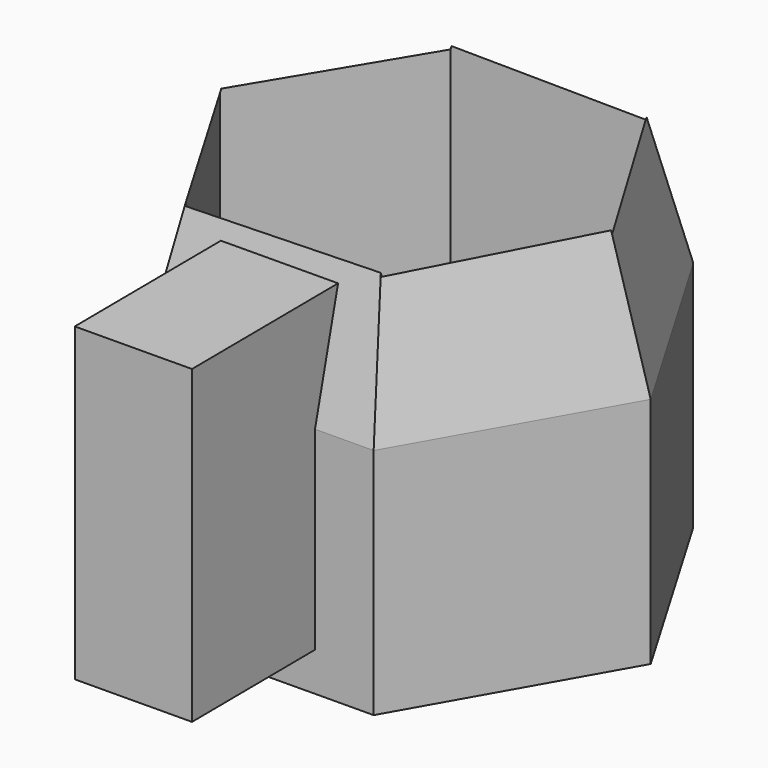
from build123d import *

# Parameters (mm, degrees)
F1_DEPTH     = 50
F3_DEPTH     = 45
F4_W         = 15
F4_H         = 40
F5_DEPTH     = 20
F6_T1_DEPTH  = 133.8850999909
F6_T3_DEPTH  = 133.8850999909
F6_T5_DEPTH  = 133.8850999909
F6_T10_DEPTH = 133.8850999909
F6_T15_DEPTH = 133.8850999909
F6_T20_DEPTH = 133.8850999909
F6_T25_DEPTH = 133.8850999909
F6_T30_DEPTH = 133.8850999909


# Not quite as in the source:
# - a fillet or chamfer that OpenCascade refuses, or shapes differently, is made with other operations: its cross-section is extruded or revolved along the edge and cut away or added


with BuildPart() as f1:
    # F0 (on Top) → F1 (new body)
    with BuildSketch(Plane.XY):
        Polygon((29.9990277389, 0.2415258118), (14.7903463808, 26.1006830166), (-15.2086813581, 25.8591572049), (-29.9990277389, -0.2415258118), (-14.7903463808, -26.1006830166), (15.2086813581, -25.8591572049), align=None)
    extrude(amount=F1_DEPTH)

    # F2 (on face) → F3 (cut)
    with BuildSketch(Plane.XY.offset(50)):
        Polygon((24.9981357174, 0.3053041981), (12.2346666673, 21.8016726776), (-12.7634690502, 21.4963684795), (-24.9981357174, -0.3053041981), (-12.2346666673, -21.8016726776), (12.7634690502, -21.4963684795), align=None)
    extrude(amount=-F3_DEPTH, mode=Mode.SUBTRACT)

    # F4 (on face) → F5 (join)
    with BuildSketch(Plane(origin=(0.2091674886, -25.9799201108, 0), x_dir=(0.9999675913, 0.0080508604, 0), z_dir=(0.0080508604, -0.9999675913, 0))):
        with Locations((0, 25)):
            Rectangle(F4_W, F4_H)
    extrude(amount=F5_DEPTH)

    # F6: chamfer of 20 x 5 on 6 edges, made by hand

    # F6_s2 → F6_t1 (cut)
    with BuildSketch(Plane(origin=(33.0034500683, 58.2415425919, 0), x_dir=(0, 0, 1), z_dir=(-0.493011546, -0.8700227672, 0))):
        Polygon((50, 20.9807621135), (30, 25.9807621135), (50, 25.9807621135), align=None)
    extrude(amount=F6_T1_DEPTH, mode=Mode.SUBTRACT)

    # F6_s4 → F6_t3 (cut)
    with BuildSketch(Plane(origin=(66.9403804743, 0.5389451243, 0), x_dir=(0, 0, 1), z_dir=(-0.9999675913, -0.0080508604, 0))):
        Polygon((50, 20.9807621135), (30, 25.9807621135), (50, 25.9807621135), align=None)
    extrude(amount=F6_T3_DEPTH, mode=Mode.SUBTRACT)

    # F6_s6 → F6_t5 (cut)
    with BuildSketch(Plane(origin=(33.936930406, -57.7025974676, 0), x_dir=(0, 0, 1), z_dir=(-0.5069560453, 0.8619719068, 0))):
        Polygon((30, 25.9807621135), (50, 20.9807621135), (50, 25.9807621135), align=None)
    extrude(amount=F6_T5_DEPTH, mode=Mode.SUBTRACT)


with BuildPart() as f6_tool8:
    # F6_s9 → F6_t10 (new body)
    with BuildSketch(Plane(origin=(-33.0034500683, -58.2415425919, 0), x_dir=(0, 0, 1), z_dir=(0.493011546, 0.8700227672, 0))):
        Polygon((30, 25.9807621135), (50, 20.9807621135), (50, 25.9807621135), align=None)
    extrude(amount=F6_T10_DEPTH)

    split(bisect_by=Plane(origin=(7.4997569347, 0.0603814529, 0), x_dir=(0, 0, 1), z_dir=(0.9999675913, 0.0080508604, 0)), keep=Keep.TOP)


with BuildPart() as f1_1:
    add(f1.part)

    # F6_t7: cut F6_tool8
    add(f6_tool8.part, mode=Mode.SUBTRACT)


with BuildPart() as f6_tool13:
    # F6_s14 → F6_t15 (new body)
    with BuildSketch(Plane(origin=(-66.9403804743, -0.5389451243, 0), x_dir=(0, 0, 1), z_dir=(0.9999675913, 0.0080508604, 0))):
        Polygon((30, 25.9807621135), (50, 20.9807621135), (50, 25.9807621135), align=None)
    extrude(amount=F6_T15_DEPTH)

    split(bisect_by=Plane(origin=(-7.4997569347, -0.0603814529, 0), x_dir=(0, 0, 1), z_dir=(-0.9999675913, -0.0080508604, 0)), keep=Keep.TOP)


with BuildPart() as f1_2:
    add(f1_1.part)

    # F6_t12: cut F6_tool13
    add(f6_tool13.part, mode=Mode.SUBTRACT)


with BuildPart() as f6_tool18:
    # F6_s19 → F6_t20 (new body)
    with BuildSketch(Plane(origin=(-66.9403804743, -0.5389451243, 0), x_dir=(0, 0, 1), z_dir=(0.9999675913, 0.0080508604, 0))):
        Polygon((30, 25.9807621135), (50, 20.9807621135), (50, 25.9807621135), align=None)
    extrude(amount=F6_T20_DEPTH)

    split(bisect_by=Plane.XY.offset(45), keep=Keep.TOP)


with BuildPart() as f1_3:
    add(f1_2.part)

    # F6_t17: cut F6_tool18
    add(f6_tool18.part, mode=Mode.SUBTRACT)


with BuildPart() as f6_tool23:
    # F6_s24 → F6_t25 (new body)
    with BuildSketch(Plane(origin=(-66.9403804743, -0.5389451243, 0), x_dir=(0, 0, 1), z_dir=(0.9999675913, 0.0080508604, 0))):
        Polygon((30, 25.9807621135), (50, 20.9807621135), (50, 25.9807621135), align=None)
    extrude(amount=F6_T25_DEPTH)

    split(bisect_by=Plane(origin=(7.4997569347, 0.0603814529, 0), x_dir=(0, 0, 1), z_dir=(0.9999675913, 0.0080508604, 0)), keep=Keep.TOP)


with BuildPart() as f1_4:
    add(f1_3.part)

    # F6_t22: cut F6_tool23
    add(f6_tool23.part, mode=Mode.SUBTRACT)


with BuildPart() as f6_tool28:
    # F6_s29 → F6_t30 (new body)
    with BuildSketch(Plane(origin=(-33.936930406, 57.7025974676, 0), x_dir=(0, 0, 1), z_dir=(0.5069560453, -0.8619719068, 0))):
        Polygon((50, 20.9807621135), (30, 25.9807621135), (50, 25.9807621135), align=None)
    extrude(amount=F6_T30_DEPTH)

    split(bisect_by=Plane(origin=(-7.4997569347, -0.0603814529, 0), x_dir=(0, 0, 1), z_dir=(-0.9999675913, -0.0080508604, 0)), keep=Keep.TOP)


with BuildPart() as f1_5:
    add(f1_4.part)

    # F6_t27: cut F6_tool28
    add(f6_tool28.part, mode=Mode.SUBTRACT)


solid = f1_5.part
